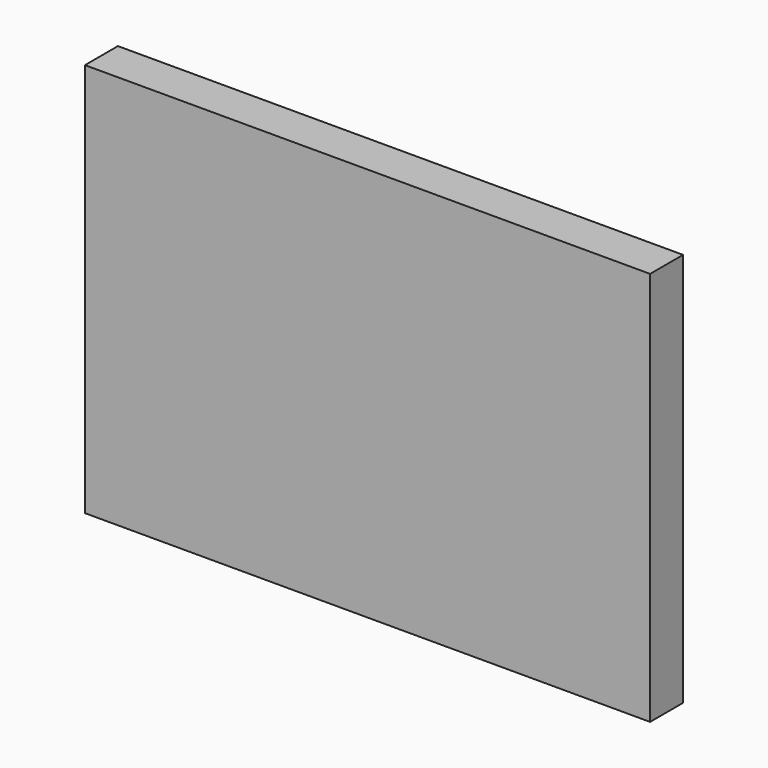
from build123d import *

# Parameters (mm, degrees)
F0_W     = 609.6
F0_H     = 406.4
F1_DEPTH = 9.525
F2_W     = 9.525
F2_H     = 406.4
F3_DEPTH = 25.4
F4_W     = 600.075
F4_H     = 406.4
F4_W_2   = 9.525
F5_DEPTH = 9.525
F6_W     = 609.6
F6_H     = 44.45
F7_DEPTH = 9.525
F8_W     = 609.6
F8_H     = 44.45
F9_DEPTH = 9.525


# Not quite as in the source:
# - a length typed as a fraction of an inch, garbled in the dataset ("3 / 203.2 mm" for 3/8 in), is restored


with BuildPart() as f1:
    # F0 (on Front) → F1 (new body)
    with BuildSketch(Plane.XZ):
        Rectangle(F0_W, F0_H)
    extrude(amount=F1_DEPTH)

    # F2 (on face) → F3 (join)
    with BuildSketch(Plane(origin=(0, 0, 0), x_dir=(-1, 0, 0), z_dir=(0, 1, 0))):
        with Locations((-300.0375, 0)):
            Rectangle(F2_W, F2_H)
        with Locations((300.0375, 0)):
            Rectangle(F2_W, F2_H)
    extrude(amount=F3_DEPTH)

    # F4 (on face) → F5 (join)
    with BuildSketch(Plane(origin=(0, 25.4, 0), x_dir=(-1, 0, 0), z_dir=(0, 1, 0))):
        with Locations((4.7625, 0)):
            Rectangle(F4_W, F4_H)
        with Locations((-300.0375, 0)):
            Rectangle(F4_W_2, F4_H)
    extrude(amount=F5_DEPTH)

    # F6 (on face) → F7 (join)
    with BuildSketch(Plane(origin=(0, 0, -203.2), x_dir=(1, 0, 0), z_dir=(0, 0, -1))):
        with Locations((0, -12.7)):
            Rectangle(F6_W, F6_H)
    extrude(amount=F7_DEPTH)

    # F8 (on face) → F9 (join)
    with BuildSketch(Plane.XY.offset(203.2)):
        with Locations((0, 12.7)):
            Rectangle(F8_W, F8_H)
    extrude(amount=F9_DEPTH)


solid = f1.part
